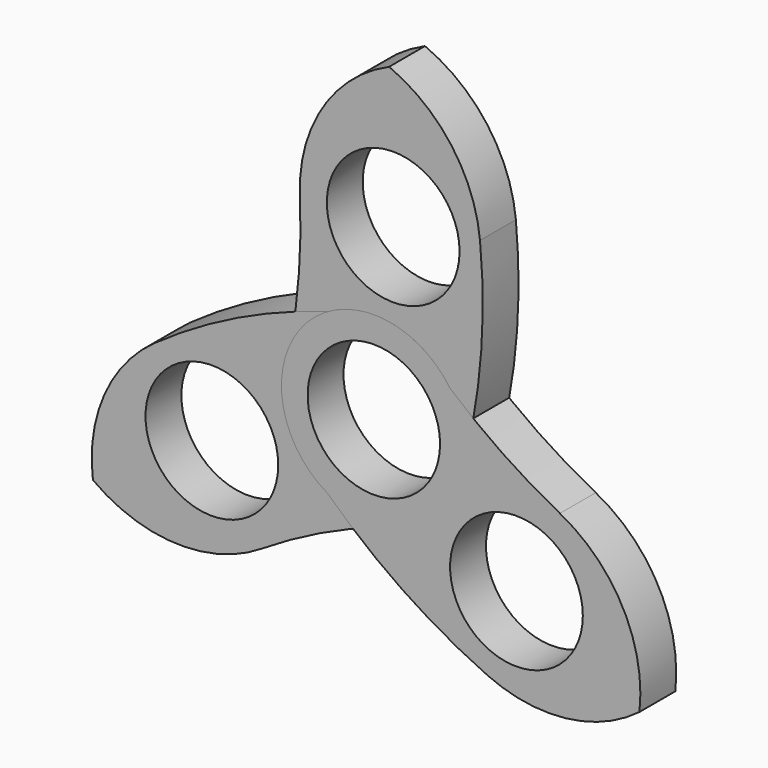
from build123d import *

# Parameters (mm, degrees)
F0_R        = 11.0769688659
F0_R_2      = 11.0998832092
F1_DEPTH    = 7.5
F2_T1_DEPTH = 123.9785226838
F2_T3_DEPTH = 155.0327099632
F3_ANGLE    = 120
F4_ANGLE    = 120


# Not quite as in the source:
# - a fillet or chamfer that OpenCascade refuses, or shapes differently, is made with other operations: its cross-section is extruded or revolved along the edge and cut away or added


with BuildPart() as f1:
    # F0 (on Front) → F1 (new body)
    with BuildSketch(Plane.XZ):
        with BuildLine():
            ThreePointArc((-13.9513406484, 6.6547180524), (-14.6452946637, 3.3140131723), (-15.4572047358, 0))
            ThreePointArc((-15.4572047358, 0), (0, -15.4572047358), (15.4572047358, 0))
            ThreePointArc((15.4572047358, 0), (3.4114842447, 15.0760390519), (-13.9513406484, 6.6547180524))
        make_face()
        Circle(F0_R, mode=Mode.SUBTRACT)
        with BuildLine():
            ThreePointArc((-13.9513406484, 6.6547180524), (-15.0760390519, 3.4114842447), (-15.4572047358, 0))
            ThreePointArc((-15.4572047358, 0), (-14.6452946637, 3.3140131723), (-13.9513406484, 6.6547180524))
        make_face()
        with BuildLine():
            ThreePointArc((-13.9513406484, 6.6547180524), (3.4114842447, 15.0760390519), (15.4572047358, 0))
            ThreePointArc((15.4572047358, 0), (18.0931544378, 27.6505048351), (12.71412801, 54.9005456269))
            Line((12.71412801, 54.9005456269), (-17.0979183167, 54.6581670642))
            ThreePointArc((-17.0979183167, 54.6581670642), (-12.4776470598, 30.856169183), (-13.9513406484, 6.6547180524))
        make_face()
        with Locations((3.2386614475, 29.418149963)):
            Circle(F0_R_2, mode=Mode.SUBTRACT)
    extrude(amount=F1_DEPTH)

    # F2: fillet of radius 25 on 2 edges, made by hand

    # F2_s2 → F2_t1 (cut)
    with BuildSketch(Plane.XZ.offset(-58.2392613419)):
        with BuildLine():
            ThreePointArc((17.7615448349, 32.1582187174), (9.6039148969, 48.320024448), (-7.3243232893, 54.7376285641))
            Line((-7.3243232893, 54.7376285641), (12.71412801, 54.9005456269))
            ThreePointArc((12.71412801, 54.9005456269), (15.9292404232, 43.6828319137), (17.7615448349, 32.1582187174))
        make_face()
    extrude(amount=F2_T1_DEPTH, mode=Mode.SUBTRACT)

    # F2_s4 → F2_t3 (cut)
    with BuildSketch(Plane.XZ.offset(-73.7663549816)):
        with BuildLine():
            ThreePointArc((12.4076485255, 54.8980538806), (-5.5218599437, 47.1094324519), (-12.3648585003, 28.7981444452))
            ThreePointArc((-12.3648585003, 28.7981444452), (-13.8444319039, 41.8904919697), (-17.0979183167, 54.6581670642))
            Line((-17.0979183167, 54.6581670642), (12.4076485255, 54.8980538806))
        make_face()
    extrude(amount=F2_T3_DEPTH, mode=Mode.SUBTRACT)


with BuildPart() as f3_1:
    # F3: copy of F1
    add(f1.part.rotate(Axis((0, -7.5, 0), (0, -1, 0)), F3_ANGLE))


with BuildPart() as f4_1:
    # F4: copy of F3_1
    add(f3_1.part.rotate(Axis((0, -7.5, 0), (0, -1, 0)), F4_ANGLE))


solid = Compound([f1.part, f3_1.part, f4_1.part])
